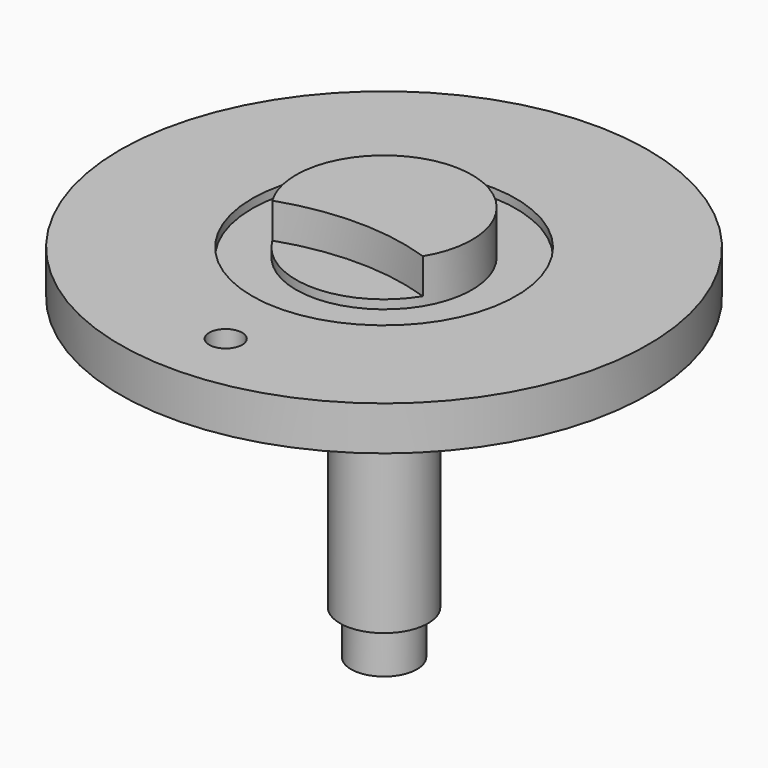
from build123d import *

# Parameters (mm, degrees)
F3_DEPTH = 25.4
F5_D     = 9.525


# Not quite as in the source:
# - a length typed as a fraction of an inch, garbled in the dataset ("3 / 203.2 mm" for 3/8 in), is restored


with BuildPart() as f1:
    # F0 (on Front) → F1 (revolve)
    with BuildSketch(Plane.XZ):
        Polygon((0, -114.3), (0, 0), (-25.4, 0), (-25.4, -12.7), (-38.1, -12.7), (-38.1, -10.16), (-76.2, -10.16), (-76.2, -22.86), (-28.575, -22.86), (-28.575, -25.4), (-12.7, -25.4), (-12.7, -101.6), (-9.525, -101.6), (-9.525, -114.3), align=None)
    revolve(axis=Axis((0, 0, -53.3123221248), (0, 0, -1)))

    # F2 (on face) → F3 (cut)
    with BuildSketch(Plane.XY.offset(-10.16)):
        with BuildLine():
            ThreePointArc((-33.332184286, -18.4546875), (0, -38.1), (33.332184286, -18.4546875))
            ThreePointArc((33.332184286, -18.4546875), (0, -9.525), (-33.332184286, -18.4546875))
        make_face()
    extrude(amount=F3_DEPTH, mode=Mode.SUBTRACT)

    # F5 (through all)
    with Locations(Plane.XY.offset(-10.16)):
        with Locations((0, -57.15)):
            Hole(F5_D / 2)


solid = f1.part
